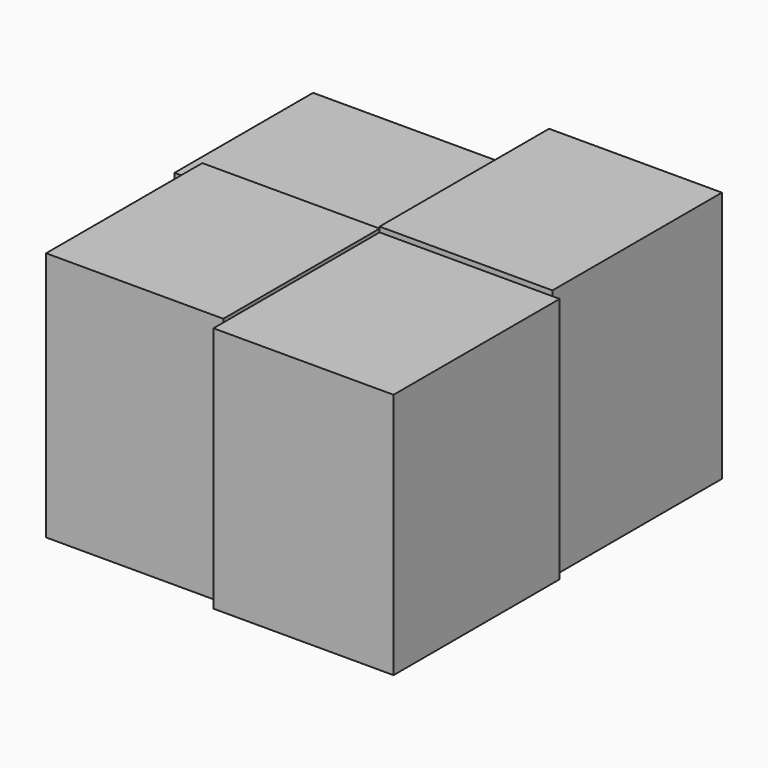
from build123d import *

# Parameters (mm, degrees)
F2_W     = 55.866792798
F2_H     = 47.1940785646
F3_DEPTH = 63.3490812033
F4_W     = 49.0447096527
F4_H     = 56.554261595
F5_DEPTH = 67.2358740121
F6_W     = 47.0842570066
F6_H     = 57.6928332448
F7_DEPTH = 68.6365682632
F8_W     = 48.2916012406
F8_H     = 53.1796514988
F9_DEPTH = 68.1448299438


# Not quite as in the source:
# - the program builds the solid bodies; features that only make, move or delete a surface that nothing else refers to are left out


with BuildPart() as f3:
    # F2 (on Top) → F3 (new body)
    with BuildSketch(Plane.XY):
        with Locations((-27.933396399, 23.5970392823)):
            Rectangle(F2_W, F2_H)
    extrude(amount=F3_DEPTH)


with BuildPart() as f5:
    # F4 (on Top) → F5 (new body)
    with BuildSketch(Plane.XY):
        with Locations((24.5223548263, -28.2771307975)):
            Rectangle(F4_W, F4_H)
    extrude(amount=F5_DEPTH)


with BuildPart() as f7:
    # F6 (on Top) → F7 (new body)
    with BuildSketch(Plane.XY):
        with Locations((23.5421285033, 28.8464166224)):
            Rectangle(F6_W, F6_H)
    extrude(amount=F7_DEPTH)


with BuildPart() as f9:
    # F8 (on Top) → F9 (new body)
    with BuildSketch(Plane.XY):
        with Locations((-24.1458006203, -26.5898257494)):
            Rectangle(F8_W, F8_H)
    extrude(amount=F9_DEPTH)


solid = Compound([f3.part, f5.part, f7.part, f9.part])
